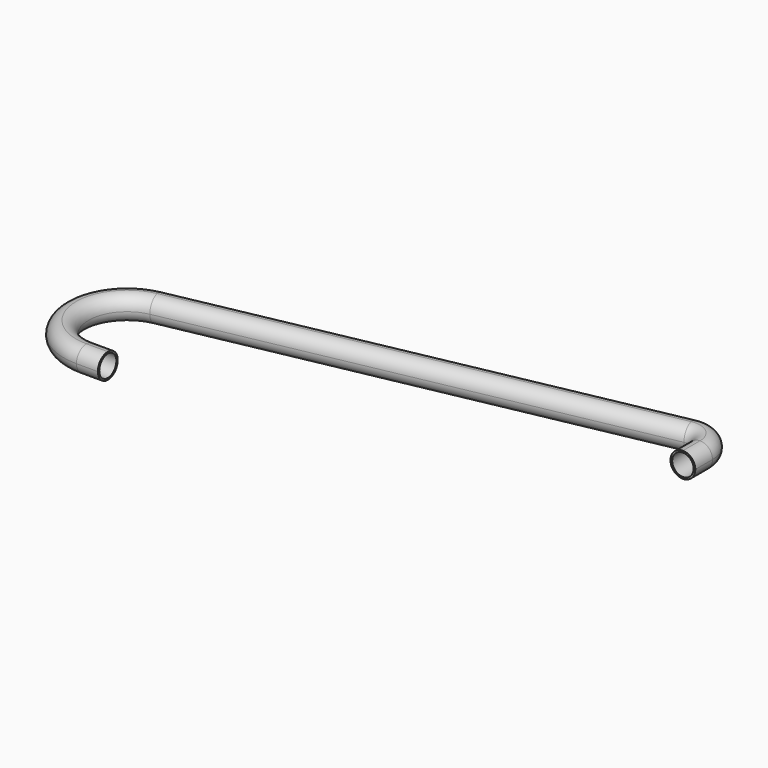
from build123d import *

# Parameters (mm, degrees)
F1_W = 3.683
F1_H = 3.683
F1_R = 1.5875
F3_R = 1.84149


# Not quite as in the source:
# - a fillet or chamfer is up to 0.001 mm smaller than in the source, because OpenCascade refuses the exact size


with BuildPart() as f2:
    # F2: sweep along a path in F0
    with BuildLine(Plane.XY) as f2_path:
        Line((0, 0), (0, 3.175))
        ThreePointArc((0, 3.175), (-1.1601260804, 5.6287538769), (-3.7926980084, 6.289333664))
        Line((-3.7926980084, 6.289333664), (-72.1618614389, -7.2710296886))
        ThreePointArc((-72.1618614389, -7.2710296886), (-78.2061381687, -15.413767246), (-70.6931784, -22.225))
        Line((-70.6931784, -22.225), (-67.5181784, -22.225))
    # F1 (on Front) → F2 (sweep)
    with BuildSketch(Plane.XZ):
        Rectangle(F1_W, F1_H)
        Circle(F1_R, mode=Mode.SUBTRACT)
    sweep(path=f2_path.line)

    # F3 (radius 1.8415 in the source; OpenCascade refuses exactly that, so slightly less here)
    f3_edges = [f2.edges().sort_by_distance(p)[0] for p in [
        (-37.619015, -2.297162, 1.8415),
        (-37.619015, -2.297162, -1.8415),
        (-38.335545, 1.315466, 1.8415),
        (-38.335545, 1.315466, -1.8415),
    ]]
    fillet(f3_edges, radius=F3_R)


solid = f2.part
